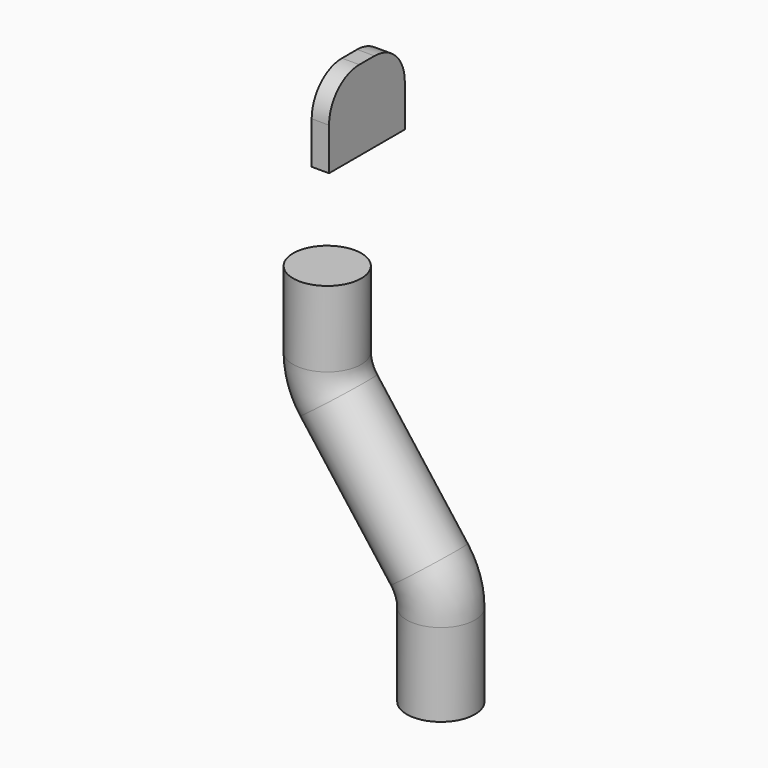
from build123d import *

# Parameters (mm, degrees)
F0_R      = 9
F3_W      = 4.5837214408
F3_H      = 21.1799524822
F4_DEPTH  = 12.5
F8_R      = 6
F9_DEPTH  = 10
F10_R     = 5.88688452
F11_DEPTH = 25
F12_R     = 10


# Not quite as in the source:
# - the program builds the solid bodies; features that only make, move or delete a surface that nothing else refers to are left out


with BuildPart() as f2:
    # F2: sweep along a path in F1
    with BuildLine(Plane.XZ) as f2_path:
        Line((0, 0), (0, 21.9242861825))
        ThreePointArc((0, 21.9242861825), (-0.7825412605, 26.7059037947), (-3.0485155987, 30.9886129972))
        Line((-3.0485155987, 30.9886129972), (-26.9514844013, 62.505124331))
        ThreePointArc((-26.9514844013, 62.505124331), (-29.2174587395, 66.7878335335), (-30, 71.5694511458))
        Line((-30, 71.5694511458), (-30, 91.5694511458))
    # F0 (on Top) → F2 (sweep)
    with BuildSketch(Plane.XY):
        Circle(F0_R)
    sweep(path=f2_path.line)

    # F8 (on Top) → F9 (cut)
    with BuildSketch(Plane.XY):
        Circle(F8_R)
    extrude(amount=F9_DEPTH, mode=Mode.SUBTRACT)

    # F10 (on face) → F11 (cut)
    with BuildSketch(Plane.YZ.offset(-19.5183108238)):
        with Locations((0, 164.4262522459)):
            Circle(F10_R)
    extrude(amount=-F11_DEPTH, mode=Mode.SUBTRACT)


with BuildPart() as f4:
    # F3 (on Front) → F4 (new body, symmetric)
    with BuildSketch(Plane.XZ):
        with Locations((-21.8101715442, 132.1594273869)):
            Rectangle(F3_W, F3_H)
    extrude(amount=F4_DEPTH, both=True)

    # F12
    f12_edges = [f4.edges().sort_by_distance(p)[0] for p in [
        (-21.810172, -12.5, 142.749404),
        (-21.810172, 12.5, 142.749404),
    ]]
    fillet(f12_edges, radius=F12_R)


solid = Compound([f2.part, f4.part])
